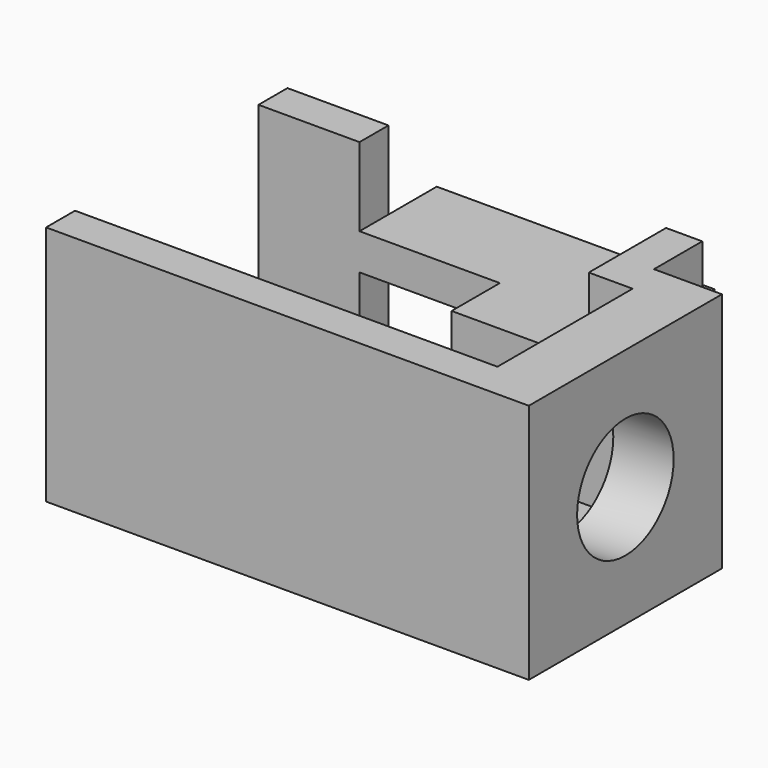
from build123d import *

# Parameters (mm, degrees)
F0_W      = 40
F0_H      = 20
F1_DEPTH  = 10
F3_W      = 35
F3_H      = 3
F4_DEPTH  = 10
F5_W      = 23
F5_H      = 3
F6_DEPTH  = 6.5
F7_W      = 23
F7_H      = 3
F8_DEPTH  = 5
F9_DEPTH  = 10
F10_DEPTH = 35
F11_DEPTH = 40
F12_DEPTH = 35
F13_DEPTH = 40
F14_DEPTH = 35
F15_W     = 20
F15_H     = 17
F16_DEPTH = 5


with BuildPart() as f1:
    # F0 (on Top) → F1 (new body)
    with BuildSketch(Plane.XY):
        Rectangle(F0_W, F0_H)
    extrude(amount=F1_DEPTH)

    # F3 (on face) → F4 (join)
    with BuildSketch(Plane.XY.offset(10)):
        Polygon((20, -10), (20, 10), (15, 10), (15, 7), (15, -7), (15, -10), align=None)
        with Locations((-2.5, 8.5)):
            Rectangle(F3_W, F3_H)
        with Locations((-2.5, -8.5)):
            Rectangle(F3_W, F3_H)
    extrude(amount=F4_DEPTH)

    # F5 (on face) → F6 (cut)
    with BuildSketch(Plane.XY.offset(20)):
        with Locations((-0.1296941414, 8.5)):
            Rectangle(F5_W, F5_H)
    extrude(amount=-F6_DEPTH, mode=Mode.SUBTRACT)

    # F7 (on face) → F8 (join)
    with BuildSketch(Plane(origin=(0, 10, 0), x_dir=(-1, 0, 0), z_dir=(0, 1, 0))):
        with Locations((0.1296941414, 12)):
            Rectangle(F7_W, F7_H)
        Polygon((-11.3703058586, 10.5), (-11.3703058586, 13.5), (-11.3703058586, 20), (-14.3703058586, 20), (-14.3703058586, 10.5), align=None)
        Polygon((11.6296941414, 20), (11.6296941414, 13.5), (11.6296941414, 10.5), (11.6296941414, 0), (20, 0), (20, 20), align=None)
    extrude(amount=F8_DEPTH)

    # F7 (on face) → F9 (join)
    with BuildSketch(Plane(origin=(0, 10, 0), x_dir=(-1, 0, 0), z_dir=(0, 1, 0))):
        with Locations((0.1296941414, 12)):
            Rectangle(F7_W, F7_H)
    extrude(amount=F9_DEPTH)

    # F2 (on face) → F10 (cut)
    with BuildSketch(Plane(origin=(-20, 0, 0), x_dir=(0, -1, 0), z_dir=(-1, 0, 0))):
        with BuildLine():
            Line((-5, 10), (-7, 10))
            ThreePointArc((-7, 10), (-4.9497474683, 5.0502525317), (0, 3))
            Line((0, 3), (0, 5))
            ThreePointArc((0, 5), (-3.5355339059, 6.4644660941), (-5, 10))
        make_face()
        with BuildLine():
            ThreePointArc((0, 5), (3.5355339059, 6.4644660941), (5, 10))
            Line((5, 10), (0, 10))
            Line((0, 10), (0, 5))
        make_face()
    extrude(amount=-F10_DEPTH, mode=Mode.SUBTRACT)

    # F2 (on face) → F11 (cut)
    with BuildSketch(Plane(origin=(-20, 0, 0), x_dir=(0, -1, 0), z_dir=(-1, 0, 0))):
        with BuildLine():
            Line((0, 10), (5, 10))
            ThreePointArc((5, 10), (0, 15), (-5, 10))
            Line((-5, 10), (0, 10))
        make_face()
        with BuildLine():
            ThreePointArc((0, 5), (3.5355339059, 6.4644660941), (5, 10))
            Line((5, 10), (0, 10))
            Line((0, 10), (0, 5))
        make_face()
        with BuildLine():
            Line((0, 10), (-5, 10))
            ThreePointArc((-5, 10), (-3.5355339059, 6.4644660941), (0, 5))
            Line((0, 5), (0, 10))
        make_face()
    extrude(amount=-F11_DEPTH, mode=Mode.SUBTRACT)

    # F2 (on face) → F12 (cut)
    with BuildSketch(Plane(origin=(-20, 0, 0), x_dir=(0, -1, 0), z_dir=(-1, 0, 0))):
        with BuildLine():
            Line((0, 10), (-5, 10))
            ThreePointArc((-5, 10), (-3.5355339059, 6.4644660941), (0, 5))
            Line((0, 5), (0, 10))
        make_face()
        with BuildLine():
            Line((-5, 10), (-7, 10))
            ThreePointArc((-7, 10), (-4.9497474683, 5.0502525317), (0, 3))
            Line((0, 3), (0, 5))
            ThreePointArc((0, 5), (-3.5355339059, 6.4644660941), (-5, 10))
        make_face()
        with BuildLine():
            ThreePointArc((0, 3), (-4.9497474683, 5.0502525317), (-7, 10))
            Line((-7, 10), (-7, 3))
            Line((-7, 3), (0, 3))
        make_face()
    extrude(amount=-F12_DEPTH, mode=Mode.SUBTRACT)

    # F2 (on face) → F13 (cut)
    with BuildSketch(Plane(origin=(-20, 0, 0), x_dir=(0, -1, 0), z_dir=(-1, 0, 0))):
        with BuildLine():
            Line((0, 10), (-5, 10))
            ThreePointArc((-5, 10), (-3.5355339059, 6.4644660941), (0, 5))
            Line((0, 5), (0, 10))
        make_face()
    extrude(amount=-F13_DEPTH, mode=Mode.SUBTRACT)

    # F2 (on face) → F14 (cut)
    with BuildSketch(Plane(origin=(-20, 0, 0), x_dir=(0, -1, 0), z_dir=(-1, 0, 0))):
        with BuildLine():
            ThreePointArc((0, 3), (4.9497474683, 5.0502525317), (7, 10))
            Line((7, 10), (5, 10))
            ThreePointArc((5, 10), (3.5355339059, 6.4644660941), (0, 5))
            Line((0, 5), (0, 3))
        make_face()
    extrude(amount=-F14_DEPTH, mode=Mode.SUBTRACT)

    # F15 (on face) → F16 (cut)
    with BuildSketch(Plane.XZ.offset(-7)):
        with Locations((-10, 11.5)):
            Rectangle(F15_W, F15_H)
    extrude(amount=-F16_DEPTH, mode=Mode.SUBTRACT)


solid = f1.part
